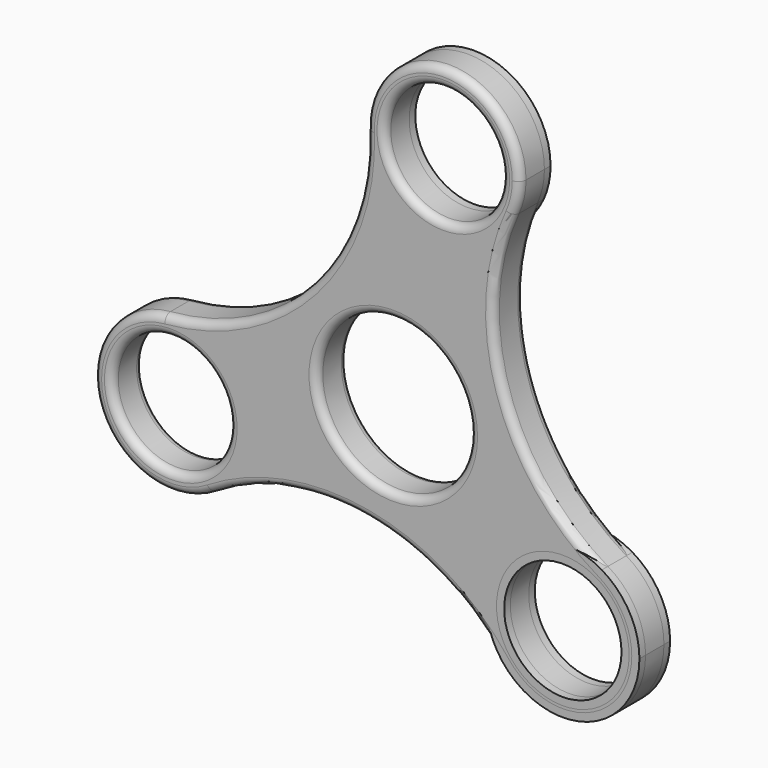
from build123d import *

# Parameters (mm, degrees)
F0_R     = 38.9001
F1_DEPTH = 25.4
F2_R     = 36.0475223941
F3_DEPTH = 25.4
F0_R_2   = 50.8
F0_R_3   = 38.9057287441
F4_DEPTH = 25.4
F5_R     = 5.08
F5_2_R   = 5.08


# Not quite as in the source:
# - a feature names something its author has since deleted; it is built from what else it names


with BuildPart() as f1:
    # F0 (on Front) → F1 (new body)
    with BuildSketch(Plane.XZ):
        with BuildLine():
            ThreePointArc((-9.9166287314, 131.8270411846), (31.0228103029, 83.8985370579), (87.088225593, 112.705626196))
            ThreePointArc((87.088225593, 112.705626196), (90.4944953008, 122.9783307664), (91.6473607783, 133.7394661017))
            ThreePointArc((91.6473607783, 133.7394661017), (39.8909788175, 184.5304626813), (-9.9166287314, 131.8270411846))
        make_face()
        with Locations((40.8473607783, 133.7394661017)):
            Circle(F0_R, mode=Mode.SUBTRACT)
    extrude(amount=F1_DEPTH)

    # F2 (on face) → F3 (cut)
    with BuildSketch(Plane.XZ.offset(25.4)):
        with Locations((40.8473607783, 133.7394661017)):
            Circle(F2_R)
    extrude(amount=-F3_DEPTH, mode=Mode.SUBTRACT)

    # F5
    f5_edges = [f1.edges().sort_by_distance(p)[0] for p in [
        (91.61135, -25.4, 135.651891),
        (1.947261, -25.4, 133.739466),
    ]]
    fillet(f5_edges, radius=F5_R)


with BuildPart() as f1b:
    # F0 (on Front) → F1, piece 2 (new body)
    with BuildSketch(Plane.XZ):
        with BuildLine():
            ThreePointArc((79.920546499, -149.0133307512), (136.5242408943, -165.9990439413), (170.899168766, -117.927669865))
            ThreePointArc((170.899168766, -117.927669865), (164.2215165418, -92.7511246939), (145.9441125945, -74.1934855409))
            ThreePointArc((145.9441125945, -74.1934855409), (82.0089351921, -84.3155573715), (79.920546499, -149.0133307512))
        make_face()
        with Locations((120.099168766, -117.927669865)):
            Circle(F0_R, mode=Mode.SUBTRACT)
    extrude(amount=F1_DEPTH)


with BuildPart() as f4:
    # F0 (on Front) → F4 (new body)
    with BuildSketch(Plane.XZ):
        with BuildLine():
            ThreePointArc((79.920546499, -149.0133307512), (136.5242408943, -165.9990439413), (170.899168766, -117.927669865))
            ThreePointArc((170.899168766, -117.927669865), (164.2215165418, -92.7511246939), (145.9441125945, -74.1934855409))
            ThreePointArc((145.9441125945, -74.1934855409), (82.0089351921, -84.3155573715), (79.920546499, -149.0133307512))
        make_face()
        with Locations((120.099168766, -117.927669865)):
            Circle(F0_R, mode=Mode.SUBTRACT)
        with BuildLine():
            ThreePointArc((79.920546499, -149.0133307512), (82.0089351921, -84.3155573715), (145.9441125945, -74.1934855409))
            ThreePointArc((145.9441125945, -74.1934855409), (80.7011021876, 7.9776457744), (87.088225593, 112.705626196))
            ThreePointArc((87.088225593, 112.705626196), (31.0228103029, 83.8985370579), (-9.9166287314, 131.8270411846))
            ThreePointArc((-9.9166287314, 131.8270411846), (-46.6389135841, 29.145231561), (-144.1053289729, -19.7667107809))
            ThreePointArc((-144.1053289729, -19.7667107809), (-105.309570926, -33.0421482364), (-88.8258923823, -70.5872734025))
            ThreePointArc((-88.8258923823, -70.5872734025), (-95.2870378452, -95.4327052049), (-113.0333730134, -113.9828930812))
            ThreePointArc((-113.0333730134, -113.9828930812), (-9.8361968908, -94.4819575628), (79.920546499, -149.0133307512))
        make_face()
        with Locations((7.6745930707, -23.3567503257)):
            Circle(F0_R_2, mode=Mode.SUBTRACT)
        with BuildLine():
            ThreePointArc((-9.9166287314, 131.8270411846), (31.0228103029, 83.8985370579), (87.088225593, 112.705626196))
            ThreePointArc((87.088225593, 112.705626196), (90.4944953008, 122.9783307664), (91.6473607783, 133.7394661017))
            ThreePointArc((91.6473607783, 133.7394661017), (39.8909788175, 184.5304626813), (-9.9166287314, 131.8270411846))
        make_face()
        with Locations((40.8473607783, 133.7394661017)):
            Circle(F0_R, mode=Mode.SUBTRACT)
        with BuildLine():
            ThreePointArc((-144.1053289729, -19.7667107809), (-188.2606792964, -86.5606592744), (-113.0333730134, -113.9828930812))
            ThreePointArc((-113.0333730134, -113.9828930812), (-95.2870378452, -95.4327052049), (-88.8258923823, -70.5872734025))
            ThreePointArc((-88.8258923823, -70.5872734025), (-105.309570926, -33.0421482364), (-144.1053289729, -19.7667107809))
        make_face()
        with Locations((-139.8571086664, -70.3821146693)):
            Circle(F0_R_3, mode=Mode.SUBTRACT)
    extrude(amount=F4_DEPTH)

    # F5#2
    f5_2_edges = [f4.edges().sort_by_distance(p)[0] for p in [
        (1.947261, -25.4, 133.739466),
        (158.189402, 0, -151.539782),
        (80.701102, 0, 7.977646),
        (50.671911, 0, 183.580395),
        (-46.638914, 0, 29.145232),
        (-188.260679, 0, -86.560659),
        (-9.836197, 0, -94.481958),
        (81.199069, 0, -117.92767),
        (-43.125407, 0, -23.35675),
        (1.947261, 0, 133.739466),
        (-178.762837, 0, -70.382115),
        (158.189402, -25.4, -151.539782),
        (80.701102, -25.4, 7.977646),
        (50.671911, -25.4, 183.580395),
        (-46.638914, -25.4, 29.145232),
        (-188.260679, -25.4, -86.560659),
        (-9.836197, -25.4, -94.481958),
        (81.199069, -25.4, -117.92767),
        (-43.125407, -25.4, -23.35675),
        (-178.762837, -25.4, -70.382115),
        (-9.916629, -12.7, 131.827041),
        (-144.105329, -12.7, -19.766711),
    ]]
    fillet(f5_2_edges, radius=F5_2_R)


solid = Compound([f1.part, f1b.part, f4.part])
